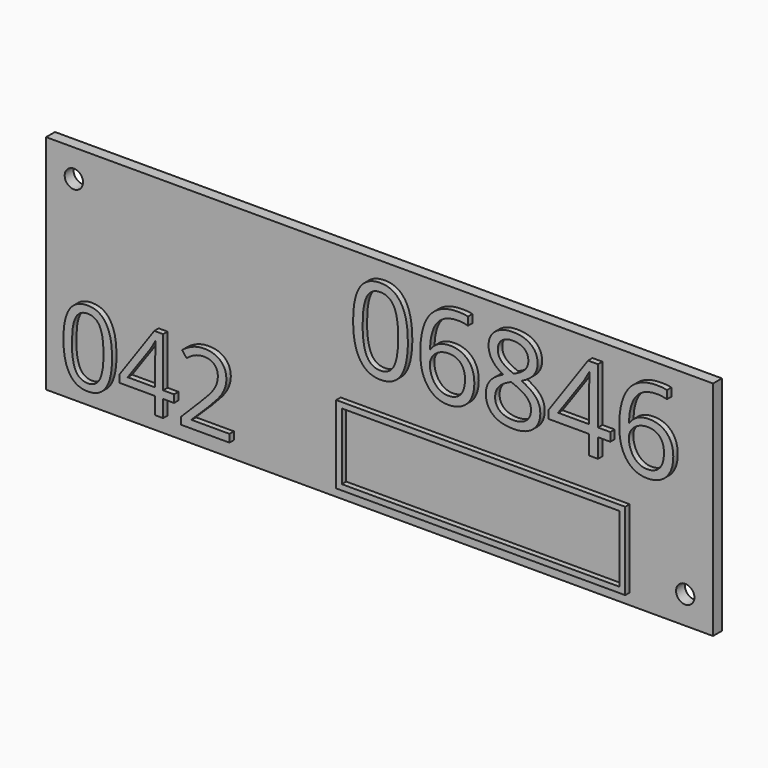
from build123d import *

# Parameters (mm, degrees)
F0_W         = 120
F0_H         = 40
F1_DEPTH     = 2
F3_D         = 3.3
F4_TEXT_SIZE = 20.871833895
F5_DEPTH     = 1
F6_TEXT_SIZE = 18.5356140827
F7_DEPTH     = 1
F8_W         = 52
F8_H         = 14
F8_W_2       = 49.99999962
F8_H_2       = 11.99999962
F9_DEPTH     = 1


# Not quite as in the source:
# - Text() gives the source's letters only with a copy of the font that has no kerning and outlines rounded to 1/6400 em; it was checked with that copy


with BuildPart() as f1:
    # F0 (on Front) → F1 (new body)
    with BuildSketch(Plane.XZ):
        Rectangle(F0_W, F0_H)
    extrude(amount=F1_DEPTH)

    # F3 (through all)
    with Locations(Plane.XZ.offset(2)):
        with Locations((-55, 15), (55, -15)):
            Hole(F3_D / 2)

    # F4 (on face) → F5 (join)
    with BuildSketch(Plane.XZ.offset(2)):
        with Locations((-5, 2)):
            Text('06846', F4_TEXT_SIZE, font='Open Sans', text_align=(TextAlign.LEFT, TextAlign.BOTTOM))
    extrude(amount=F5_DEPTH)

    # F6 (on face) → F7 (join)
    with BuildSketch(Plane.XZ.offset(2)):
        with Locations((-57, -17)):
            Text('042', F6_TEXT_SIZE, font='Open Sans', text_align=(TextAlign.LEFT, TextAlign.BOTTOM))
    extrude(amount=F7_DEPTH)

    # F8 (on face) → F9 (join)
    with BuildSketch(Plane.XZ.offset(2)):
        with Locations((19, -11)):
            Rectangle(F8_W, F8_H)
        with Locations((19, -11)):
            Rectangle(F8_W_2, F8_H_2, mode=Mode.SUBTRACT)
    extrude(amount=F9_DEPTH)


solid = f1.part
